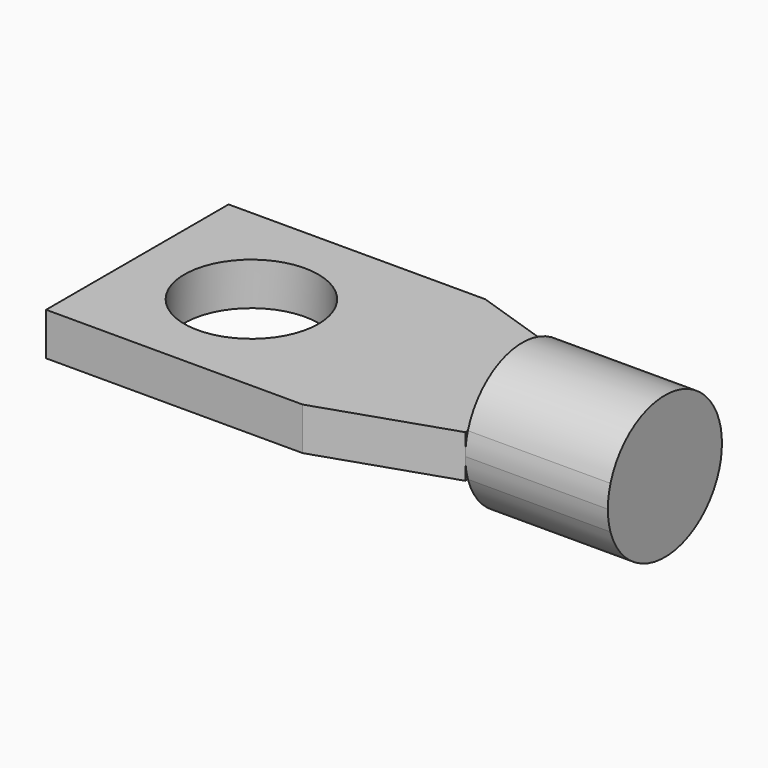
from build123d import *

# Parameters (mm, degrees)
F0_R     = 23.5
F1_DEPTH = 15
F3_DEPTH = 50


with BuildPart() as f1:
    # F0 (on Top) → F1 (new body)
    with BuildSketch(Plane.XY):
        Polygon((-90, -40), (0, -40), (45, -25), (45, 25), (0, 40), (-90, 40), align=None)
        with Locations((-50, 0)):
            Circle(F0_R, mode=Mode.SUBTRACT)
    extrude(amount=F1_DEPTH)

    # F2 (on face) → F3 (join)
    with BuildSketch(Plane.YZ.offset(45)):
        with BuildLine():
            ThreePointArc((23.8484800354, 0), (24.7104431454, 3.7060575179), (25, 7.5))
            ThreePointArc((25, 7.5), (24.7104431454, 11.2939424821), (23.8484800354, 15))
            Line((23.8484800354, 15), (-23.8484800354, 15))
            ThreePointArc((-23.8484800354, 15), (-24.7104431454, 11.2939424821), (-25, 7.5))
            ThreePointArc((-25, 7.5), (-24.7104431454, 3.7060575179), (-23.8484800354, 0))
            Line((-23.8484800354, 0), (23.8484800354, 0))
        make_face()
        with BuildLine():
            Line((-23.8484800354, 15), (23.8484800354, 15))
            ThreePointArc((23.8484800354, 15), (0, 32.5), (-23.8484800354, 15))
        make_face()
        with BuildLine():
            ThreePointArc((-23.8484800354, 0), (0, -17.5), (23.8484800354, 0))
            Line((23.8484800354, 0), (-23.8484800354, 0))
        make_face()
    extrude(amount=F3_DEPTH)


solid = f1.part
